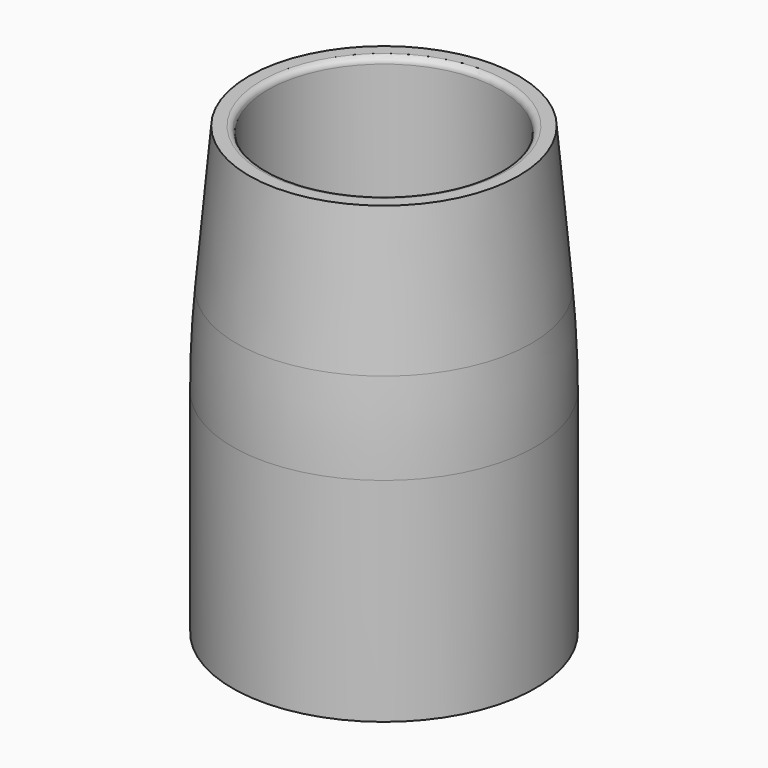
from build123d import *

# Parameters (mm, degrees)
F2_R = 0.6


# Not quite as in the source:
# - a fillet or chamfer that OpenCascade refuses, or shapes differently, is made with other operations: its cross-section is extruded or revolved along the edge and cut away or added


with BuildPart() as f1:
    # F0 (on Front) → F1 (revolve)
    with BuildSketch(Plane.XZ):
        Polygon((-14.7, 15), (-14.7, 0), (-14.7, -10), (-12.9, -10), (-12.9, 0), (-11.3, 18.2880836844), (-11.3, 33.2880836844), (-13.1, 33.2880836844), align=None)
    revolve(axis=Axis((0, 0, 16.6440418422), (0, 0, 1)))

    # F2
    f2_edges = [f1.edges().sort_by_distance(p)[0] for p in [
        (11.3, 0, 33.288084),
    ]]
    fillet(f2_edges, radius=F2_R)

    # F3: fillet of radius 100 on 1 edges, made by hand

    # F3_s1 → F3_t2 (revolve, cut)
    with BuildSketch(Plane.XZ):
        with BuildLine():
            ThreePointArc((-14.3194698092, 19.3494799839), (-14.6048221582, 14.9958444457), (-14.7, 10.6339057091))
            Line((-14.7, 10.6339057091), (-14.7, 15))
            Line((-14.7, 15), (-14.3194698092, 19.3494799839))
        make_face()
    revolve(axis=Axis((0, 0, 15), (0, 0, 1)), mode=Mode.SUBTRACT)


solid = f1.part
